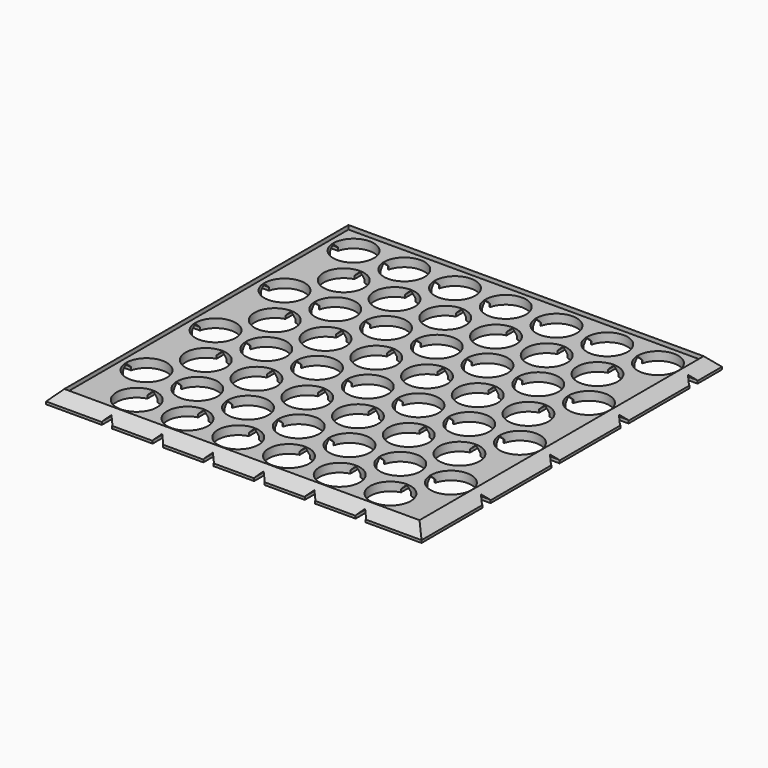
from build123d import *

# Parameters (mm, degrees)
F0_W         = 74
F0_H         = 74
F0_W_2       = 70
F0_H_2       = 70
F1_DEPTH     = 2.5
F2_DEPTH     = 1.7
F3_W         = 2
F3_H         = 80
F5_DEPTH     = 0.6
F4_W         = 80
F4_H         = 2
F6_DEPTH     = 0.6
F8_DEPTH     = 74
F10_DEPTH    = 74.001
F12_T1_DEPTH = 84.2867319519
F12_T3_DEPTH = 84.2867319519
F11_R        = 4
F13_DEPTH    = 2.501


# Not quite as in the source:
# - a fillet or chamfer that OpenCascade refuses, or shapes differently, is made with other operations: its cross-section is extruded or revolved along the edge and cut away or added


with BuildPart() as f1:
    # F0 (on Top) → F1 (new body)
    with BuildSketch(Plane.XY):
        with Locations((35, 35)):
            Rectangle(F0_W, F0_H)
        with Locations((35, 35)):
            Rectangle(F0_W_2, F0_H_2, mode=Mode.SUBTRACT)
    extrude(amount=F1_DEPTH)

    # F0 (on Top) → F2 (join)
    with BuildSketch(Plane.XY):
        with Locations((35, 35)):
            Rectangle(F0_W, F0_H)
        with Locations((35, 35)):
            Rectangle(F0_W_2, F0_H_2, mode=Mode.SUBTRACT)
        with Locations((35, 35)):
            Rectangle(F0_W_2, F0_H_2)
    extrude(amount=F2_DEPTH)

    # F3 (on Top) → F5 (cut)
    with BuildSketch(Plane.XY):
        with Locations((10, 36)):
            Rectangle(F3_W, F3_H)
        with Locations((20, 36)):
            Rectangle(F3_W, F3_H)
        with Locations((30, 36)):
            Rectangle(F3_W, F3_H)
        with Locations((40, 36)):
            Rectangle(F3_W, F3_H)
        with Locations((50, 36)):
            Rectangle(F3_W, F3_H)
        with Locations((60, 36)):
            Rectangle(F3_W, F3_H)
    extrude(amount=F5_DEPTH, mode=Mode.SUBTRACT)

    # F4 (on Top) → F6 (cut)
    with BuildSketch(Plane.XY):
        with Locations((36, 14)):
            Rectangle(F4_W, F4_H)
        with Locations((36, 31)):
            Rectangle(F4_W, F4_H)
        with Locations((36, 48)):
            Rectangle(F4_W, F4_H)
        with Locations((36, 65)):
            Rectangle(F4_W, F4_H)
    extrude(amount=F6_DEPTH, mode=Mode.SUBTRACT)

    # F7 (on face) → F8 (cut, through all)
    with BuildSketch(Plane.XZ.offset(2)):
        Polygon((10, 1.6), (9, 0.6), (11, 0.6), align=None)
        Polygon((21, 0.6), (20, 1.6), (19, 0.6), align=None)
        Polygon((31, 0.6), (30, 1.6), (29, 0.6), align=None)
        Polygon((41, 0.6), (40, 1.6), (39, 0.6), align=None)
        Polygon((51, 0.6), (50, 1.6), (49, 0.6), align=None)
        Polygon((61, 0.6), (60, 1.6), (59, 0.6), align=None)
    extrude(amount=-F8_DEPTH, mode=Mode.SUBTRACT)

    # F9 (on face) → F10 (cut, through all)
    with BuildSketch(Plane(origin=(-2, 0, 0), x_dir=(0, -1, 0), z_dir=(-1, 0, 0))):
        Polygon((-65, 1.6), (-66, 0.6), (-64, 0.6), align=None)
        Polygon((-47, 0.6), (-48, 1.6), (-49, 0.6), align=None)
        Polygon((-30, 0.6), (-31, 1.6), (-32, 0.6), align=None)
        Polygon((-13, 0.6), (-14, 1.6), (-15, 0.6), align=None)
    extrude(amount=-F10_DEPTH, mode=Mode.SUBTRACT)

    # F12: chamfer of 2 on 4 edges, made by hand

    # F12_s2 → F12_t1 (cut)
    with BuildSketch(Plane.XZ.offset(-77.1433659759)):
        Polygon((70, 2.5), (72, 0.5), (72, 2.5), align=None)
        Polygon((-2, 0.5), (0, 2.5), (-2, 2.5), align=None)
    extrude(amount=F12_T1_DEPTH, mode=Mode.SUBTRACT)

    # F12_s4 → F12_t3 (cut)
    with BuildSketch(Plane.YZ.offset(-7.1433659759)):
        Polygon((0, 2.5), (-2, 0.5), (-2, 2.5), align=None)
        Polygon((72, 0.5), (70, 2.5), (72, 2.5), align=None)
    extrude(amount=F12_T3_DEPTH, mode=Mode.SUBTRACT)

    # F11 (on face) → F13 (cut, through all)
    with BuildSketch(Plane.XY):
        with Locations((5, 65)):
            Circle(F11_R)
        with Locations((15, 65)):
            Circle(F11_R)
        with Locations((25, 65)):
            Circle(F11_R)
        with Locations((35, 65)):
            Circle(F11_R)
        with Locations((45, 65)):
            Circle(F11_R)
        with Locations((10, 56.3397459622)):
            Circle(F11_R)
        with Locations((20, 56.3397459622)):
            Circle(F11_R)
        with Locations((30, 56.3397459622)):
            Circle(F11_R)
        with Locations((40, 56.3397459622)):
            Circle(F11_R)
        with Locations((55, 65)):
            Circle(F11_R)
        with Locations((65, 65)):
            Circle(F11_R)
        with Locations((50, 56.3397459622)):
            Circle(F11_R)
        with Locations((60, 56.3397459622)):
            Circle(F11_R)
        with Locations((55, 48)):
            Circle(F11_R)
        with Locations((20, 39.3397459622)):
            Circle(F11_R)
        with Locations((65, 48)):
            Circle(F11_R)
        with Locations((60, 39.3397459622)):
            Circle(F11_R)
        with Locations((50, 39.3397459622)):
            Circle(F11_R)
        with Locations((30, 39.3397459622)):
            Circle(F11_R)
        with Locations((10, 39.3397459622)):
            Circle(F11_R)
        with Locations((5, 48)):
            Circle(F11_R)
        with Locations((40, 39.3397459622)):
            Circle(F11_R)
        with Locations((15, 48)):
            Circle(F11_R)
        with Locations((25, 48)):
            Circle(F11_R)
        with Locations((35, 48)):
            Circle(F11_R)
        with Locations((45, 48)):
            Circle(F11_R)
        with Locations((55, 31)):
            Circle(F11_R)
        with Locations((20, 22.3397459622)):
            Circle(F11_R)
        with Locations((65, 31)):
            Circle(F11_R)
        with Locations((60, 22.3397459622)):
            Circle(F11_R)
        with Locations((50, 22.3397459622)):
            Circle(F11_R)
        with Locations((30, 22.3397459622)):
            Circle(F11_R)
        with Locations((10, 22.3397459622)):
            Circle(F11_R)
        with Locations((5, 31)):
            Circle(F11_R)
        with Locations((40, 22.3397459622)):
            Circle(F11_R)
        with Locations((15, 31)):
            Circle(F11_R)
        with Locations((25, 31)):
            Circle(F11_R)
        with Locations((35, 31)):
            Circle(F11_R)
        with Locations((45, 31)):
            Circle(F11_R)
        with Locations((55, 14)):
            Circle(F11_R)
        with Locations((20, 5.3397459622)):
            Circle(F11_R)
        with Locations((65, 14)):
            Circle(F11_R)
        with Locations((60, 5.3397459622)):
            Circle(F11_R)
        with Locations((50, 5.3397459622)):
            Circle(F11_R)
        with Locations((30, 5.3397459622)):
            Circle(F11_R)
        with Locations((10, 5.3397459622)):
            Circle(F11_R)
        with Locations((5, 14)):
            Circle(F11_R)
        with Locations((40, 5.3397459622)):
            Circle(F11_R)
        with Locations((15, 14)):
            Circle(F11_R)
        with Locations((25, 14)):
            Circle(F11_R)
        with Locations((35, 14)):
            Circle(F11_R)
        with Locations((45, 14)):
            Circle(F11_R)
    extrude(amount=F13_DEPTH, mode=Mode.SUBTRACT)


solid = f1.part
